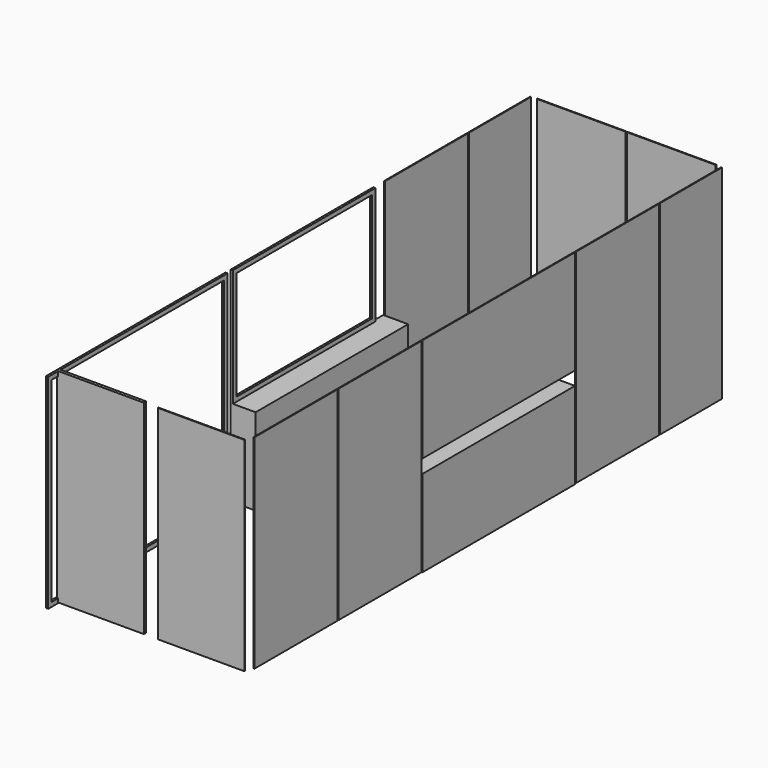
from build123d import *

# Parameters (mm, degrees)
F0_W      = 2247.9
F0_H      = 6959.6
F1_DEPTH  = 2565.4
F6_W      = 1219.2
F6_H      = 2387.6
F7_DEPTH  = 9.525
F6_W_2    = 2235.2
F6_H_2    = 1219.2
F6_W_3    = 908.05
F6_H_3    = 1016
F10_DEPTH = 292.1
F8_W      = 2628.9
F8_H      = 2393.95
F12_DEPTH = 25.4
F8_W_2    = 2089.15
F8_H_2    = 1377.95
F13_DEPTH = 292.1
F8_W_3    = 1219.2
F8_H_3    = 2387.6
F14_DEPTH = 9.525
F8_W_4    = 908.05
F9_W      = 1041.4
F9_H      = 2387.6
F15_DEPTH = 9.525
F11_W     = 1016
F11_H     = 2387.6
F16_DEPTH = 9.525
F18_DEPTH = 25.4
F19_W     = 2527.3
F19_H     = 2292.35
F20_DEPTH = 127
F21_W     = 1987.55
F21_H     = 1276.35
F22_DEPTH = 127


with BuildPart() as f1:
    # F0 (on Top) → F1 (new body)
    with BuildSketch(Plane.XY):
        with Locations((1123.95, -3479.8)):
            Rectangle(F0_W, F0_H)
    extrude(amount=F1_DEPTH)


with BuildPart() as f7:
    # F6 (on offset) → F7 (new body)
    with BuildSketch(Plane.YZ.offset(2247.9)):
        with Locations((-5022.85, 1200.15)):
            Rectangle(F6_W, F6_H)
    extrude(amount=-F7_DEPTH)


with BuildPart() as f7b:
    # F6 (on offset) → F7, piece 2 (new body)
    with BuildSketch(Plane.YZ.offset(2247.9)):
        with Locations((-3282.95, 1784.35)):
            Rectangle(F6_W_2, F6_H_2)
    extrude(amount=-F7_DEPTH)


with BuildPart() as f7c:
    # F6 (on offset) → F7, piece 3 (new body)
    with BuildSketch(Plane.YZ.offset(2247.9)):
        with Locations((-1543.05, 1200.15)):
            Rectangle(F6_W, F6_H)
    extrude(amount=-F7_DEPTH)


with BuildPart() as f7d:
    # F6 (on offset) → F7, piece 4 (new body)
    with BuildSketch(Plane.YZ.offset(2247.9)):
        with Locations((-6254.75, 1200.15)):
            Rectangle(F6_W, F6_H)
    extrude(amount=-F7_DEPTH)


with BuildPart() as f7e:
    # F6 (on offset) → F7, piece 5 (new body)
    with BuildSketch(Plane.YZ.offset(2247.9)):
        with Locations((-466.725, 1200.15)):
            Rectangle(F6_W_3, F6_H)
    extrude(amount=-F7_DEPTH)


with BuildPart() as f10:
    # F6 (on offset) → F10 (new body)
    with BuildSketch(Plane.YZ.offset(2247.9)):
        with Locations((-3282.95, 508)):
            Rectangle(F6_W_2, F6_H_3)
    extrude(amount=-F10_DEPTH)


with BuildPart() as f12:
    # F8 (on offset) → F12 (new body)
    with BuildSketch(Plane(origin=(0, 0, 0), x_dir=(0, -1, 0), z_dir=(-1, 0, 0))):
        with Locations((5791.2, 1196.975)):
            Rectangle(F8_W, F8_H)
    extrude(amount=-F12_DEPTH)

    # F19 (on face) → F20 (cut)
    with BuildSketch(Plane(origin=(0, 0, 0), x_dir=(0, -1, 0), z_dir=(-1, 0, 0))):
        with Locations((5791.2, 1196.975)):
            Rectangle(F19_W, F19_H)
    extrude(amount=-F20_DEPTH, mode=Mode.SUBTRACT)


with BuildPart() as f12b:
    # F8 (on offset) → F12, piece 2 (new body)
    with BuildSketch(Plane(origin=(0, 0, 0), x_dir=(0, -1, 0), z_dir=(-1, 0, 0))):
        with Locations((3355.975, 1704.975)):
            Rectangle(F8_W_2, F8_H_2)
    extrude(amount=-F12_DEPTH)

    # F21 (on face) → F22 (cut)
    with BuildSketch(Plane(origin=(0, 0, 0), x_dir=(0, -1, 0), z_dir=(-1, 0, 0))):
        with Locations((3355.975, 1704.975)):
            Rectangle(F21_W, F21_H)
    extrude(amount=-F22_DEPTH, mode=Mode.SUBTRACT)


with BuildPart() as f13:
    # F8 (on offset) → F13 (new body)
    with BuildSketch(Plane(origin=(0, 0, 0), x_dir=(0, -1, 0), z_dir=(-1, 0, 0))):
        Polygon((4400.55, 0), (4400.55, 1016), (2311.4, 1016), (2165.35, 1016), (2165.35, 0), align=None)
    extrude(amount=-F13_DEPTH)


with BuildPart() as f14:
    # F8 (on offset) → F14 (new body)
    with BuildSketch(Plane(origin=(0, 0, 0), x_dir=(0, -1, 0), z_dir=(-1, 0, 0))):
        with Locations((1543.05, 1200.15)):
            Rectangle(F8_W_3, F8_H_3)
    extrude(amount=-F14_DEPTH)


with BuildPart() as f14b:
    # F8 (on offset) → F14, piece 2 (new body)
    with BuildSketch(Plane(origin=(0, 0, 0), x_dir=(0, -1, 0), z_dir=(-1, 0, 0))):
        with Locations((466.725, 1200.15)):
            Rectangle(F8_W_4, F8_H_3)
    extrude(amount=-F14_DEPTH)


with BuildPart() as f15:
    # F9 (on offset) → F15 (new body)
    with BuildSketch(Plane(origin=(0, 0, 0), x_dir=(-1, 0, 0), z_dir=(0, 1, 0))):
        with Locations((-596.9, 1200.15)):
            Rectangle(F9_W, F9_H)
    extrude(amount=-F15_DEPTH)


with BuildPart() as f15b:
    # F9 (on offset) → F15, piece 2 (new body)
    with BuildSketch(Plane(origin=(0, 0, 0), x_dir=(-1, 0, 0), z_dir=(0, 1, 0))):
        with Locations((-1651, 1200.15)):
            Rectangle(F9_W, F9_H)
    extrude(amount=-F15_DEPTH)


with BuildPart() as f16:
    # F11 (on offset) → F16 (new body)
    with BuildSketch(Plane.XZ.offset(6959.6)):
        with Locations((520.7, 1200.15)):
            Rectangle(F11_W, F11_H)
    extrude(amount=-F16_DEPTH)

    # F18 (add): a face of the model
    f18_faces = [f16.faces().sort_by_distance(p)[0] for p in [
        (520.7, -6950.075, 1200.15),
    ]]
    extrude(f18_faces, amount=F18_DEPTH)


with BuildPart() as f16b:
    # F11 (on offset) → F16, piece 2 (new body)
    with BuildSketch(Plane.XZ.offset(6959.6)):
        with Locations((1701.8, 1200.15)):
            Rectangle(F11_W, F11_H)
    extrude(amount=-F16_DEPTH)


solid = Compound([f7.part, f7b.part, f7c.part, f7d.part, f7e.part, f10.part, f12.part, f12b.part, f13.part, f14.part, f14b.part, f15.part, f15b.part, f16.part, f16b.part])
